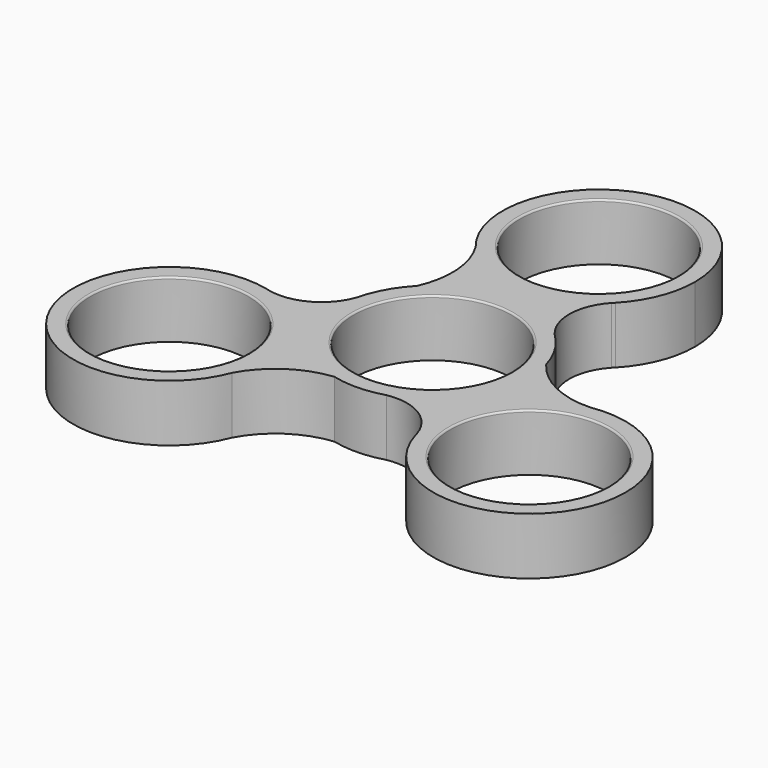
from build123d import *

# Parameters (mm, degrees)
F0_R     = 11.1
F1_DEPTH = 8
F2_R     = 0.25


# Not quite as in the source:
# - a feature of the source that left no trace in its solid (it failed there, or was rolled back) is left out


with BuildPart() as f1:
    # F0 (on Top) → F1 (new body)
    with BuildSketch(Plane.XY):
        with BuildLine():
            ThreePointArc((3.859865491, -12.9364383967), (10.8249291944, -8.0666540731), (13.5, 0))
            ThreePointArc((13.5, 0), (13.3707834369, 1.8633706782), (12.9856073653, 3.691070489))
            ThreePointArc((12.9856073653, 3.691070489), (11.5424684167, 7.0015300363), (9.2733515405, 9.8109607688))
            ThreePointArc((9.2733515405, 9.8109607688), (-0.2922686684, 13.4968358894), (-9.6893644933, 9.4003306174))
            ThreePointArc((-9.6893644933, 9.4003306174), (-11.8347370851, 6.4953058532), (-13.1332170315, 3.1254776279))
            ThreePointArc((-13.1332170315, 3.1254776279), (-11.5424684167, -7.0015300363), (-3.296242872, -13.0914011064))
            ThreePointArc((-3.296242872, -13.0914011064), (0.2922686684, -13.4968358894), (3.859865491, -12.9364383967))
        make_face()
        Circle(F0_R, mode=Mode.SUBTRACT)
        with BuildLine():
            ThreePointArc((12.9856073653, 3.691070489), (13.3707834369, 1.8633706782), (13.5, 0))
            ThreePointArc((13.5, 0), (10.8249291944, -8.0666540731), (3.859865491, -12.9364383967))
            ThreePointArc((3.859865491, -12.9364383967), (8.9875948966, -13.8732661585), (12.1902212779, -17.985982946))
            ThreePointArc((12.1902212779, -17.985982946), (13.9354582524, -7.2213929241), (23.0659975588, -1.2585494405))
            ThreePointArc((23.0659975588, -1.2585494405), (17.4140534965, -0.0296267076), (12.9856073653, 3.691070489))
        make_face()
        with BuildLine():
            ThreePointArc((-9.6893644933, 9.4003306174), (-0.2922686684, 13.4968358894), (9.2733515405, 9.8109607688))
            ThreePointArc((9.2733515405, 9.8109607688), (7.5208034785, 14.7201185786), (9.4812075043, 19.5500327774))
            ThreePointArc((9.4812075043, 19.5500327774), (-0.7138194032, 15.679157322), (-10.443062992, 20.6050145698))
            ThreePointArc((-10.443062992, 20.6050145698), (-8.6813692668, 15.0958260647), (-9.6893644933, 9.4003306174))
        make_face()
        with BuildLine():
            ThreePointArc((38.7535366191, -14.580136165), (33.9919066812, -4.2898063036), (23.0659975588, -1.2585494405))
            ThreePointArc((23.0659975588, -1.2585494405), (13.9354582524, -7.2213929241), (12.1902212779, -17.985982946))
            ThreePointArc((12.1902212779, -17.985982946), (12.2464624781, -18.1789066882), (12.297383992, -18.3733022703))
            ThreePointArc((12.297383992, -18.3733022703), (27.1695141155, -27.9434826858), (38.7535366191, -14.580136165))
        make_face()
        with Locations((25.2535366191, -14.580136165)):
            Circle(F0_R, mode=Mode.SUBTRACT)
        with BuildLine():
            ThreePointArc((-12.6229345668, -19.3464651293), (-8.7326842297, -15.066199357), (-3.296242872, -13.0914011064))
            ThreePointArc((-3.296242872, -13.0914011064), (-11.5424684167, -7.0015300363), (-13.1332170315, 3.1254776279))
            ThreePointArc((-13.1332170315, 3.1254776279), (-16.508398375, -0.8468524201), (-21.6714287822, -1.5640498314))
            ThreePointArc((-21.6714287822, -1.5640498314), (-14.5155559943, -6.3980965598), (-11.7535366191, -14.580136165))
            ThreePointArc((-11.7535366191, -14.580136165), (-11.9726645147, -17.0026216958), (-12.6229345668, -19.3464651293))
        make_face()
        with BuildLine():
            ThreePointArc((12.297383992, -18.3733022703), (12.2464624781, -18.1789066882), (12.1902212779, -17.985982946))
            ThreePointArc((12.1902212779, -17.985982946), (12.24236133, -18.1800413854), (12.297383992, -18.3733022703))
        make_face()
        with BuildLine():
            ThreePointArc((9.7630545215, 19.8364980723), (9.620163766, 19.6952009566), (9.4812075043, 19.5500327774))
            ThreePointArc((9.4812075043, 19.5500327774), (9.6231970167, 19.6922166068), (9.7630545215, 19.8364980723))
        make_face()
        with BuildLine():
            ThreePointArc((-10.443062992, 20.6050145698), (-0.7138194032, 15.679157322), (9.4812075043, 19.5500327774))
            ThreePointArc((9.4812075043, 19.5500327774), (9.620163766, 19.6952009566), (9.7630545215, 19.8364980723))
            ThreePointArc((9.7630545215, 19.8364980723), (12.5309863148, 24.1378842547), (13.5, 29.16027233))
            ThreePointArc((13.5, 29.16027233), (-4.5425020422, 41.8730877223), (-10.443062992, 20.6050145698))
        make_face()
        with Locations((0, 29.16027233)):
            Circle(F0_R, mode=Mode.SUBTRACT)
        with BuildLine():
            ThreePointArc((-22.0604385135, -1.463195802), (-37.1929755561, -20.8809137257), (-12.6229345668, -19.3464651293))
            ThreePointArc((-12.6229345668, -19.3464651293), (-11.9726645147, -17.0026216958), (-11.7535366191, -14.580136165))
            ThreePointArc((-11.7535366191, -14.580136165), (-14.5155559943, -6.3980965598), (-21.6714287822, -1.5640498314))
            ThreePointArc((-21.6714287822, -1.5640498314), (-21.8666262441, -1.5162942684), (-22.0604385135, -1.463195802))
        make_face()
        with Locations((-25.2535366191, -14.580136165)):
            Circle(F0_R, mode=Mode.SUBTRACT)
        with BuildLine():
            ThreePointArc((-22.0604385135, -1.463195802), (-21.8666262441, -1.5162942684), (-21.6714287822, -1.5640498314))
            ThreePointArc((-21.6714287822, -1.5640498314), (-21.8655583466, -1.5121752213), (-22.0604385135, -1.463195802))
        make_face()
    extrude(amount=F1_DEPTH)

    # F2
    f2_edges = [f1.edges().sort_by_distance(p)[0] for p in [
        (-11.1, 29.160272, 8),
        (-36.353537, -14.580136, 8),
        (14.153537, -14.580136, 8),
        (-11.1, 0, 8),
    ]]
    fillet(f2_edges, radius=F2_R)


solid = f1.part
